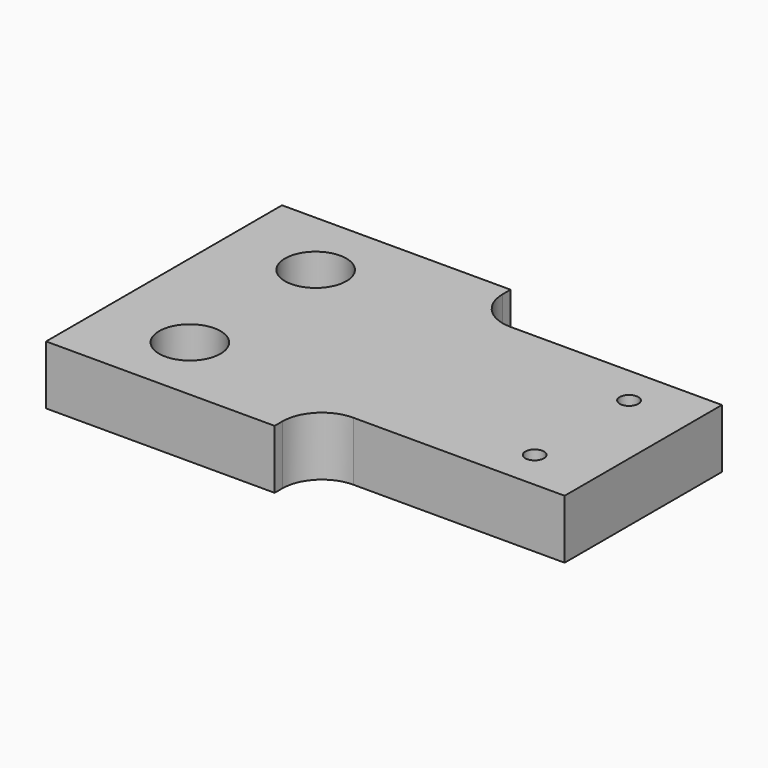
from build123d import *

# Parameters (mm, degrees)
F0_R     = 3.96875
F0_R_2   = 1.2
F1_DEPTH = 7.62
F2_R     = 5.08


with BuildPart() as f1:
    # F0 (on Top) → F1 (new body)
    with BuildSketch(Plane.XY):
        Polygon((14.76375, 19.05), (-14.76375, 19.05), (-14.76375, 12.7), (-14.76375, -12.7), (-14.76375, -19.05), (14.76375, -19.05), (14.76375, -12.7), (47.14875, -12.7), (47.14875, 12.7), (14.76375, 12.7), align=None)
        with Locations((-3.302, -10.16)):
            Circle(F0_R, mode=Mode.SUBTRACT)
        with Locations((39.21125, -7.62)):
            Circle(F0_R_2, mode=Mode.SUBTRACT)
        with Locations((-3.302, 10.16)):
            Circle(F0_R, mode=Mode.SUBTRACT)
        with Locations((39.21125, 7.62)):
            Circle(F0_R_2, mode=Mode.SUBTRACT)
    extrude(amount=F1_DEPTH)

    # F2
    f2_edges = [f1.edges().sort_by_distance(p)[0] for p in [
        (14.76375, -12.7, 3.81),
        (14.76375, 12.7, 3.81),
    ]]
    fillet(f2_edges, radius=F2_R)


solid = f1.part
